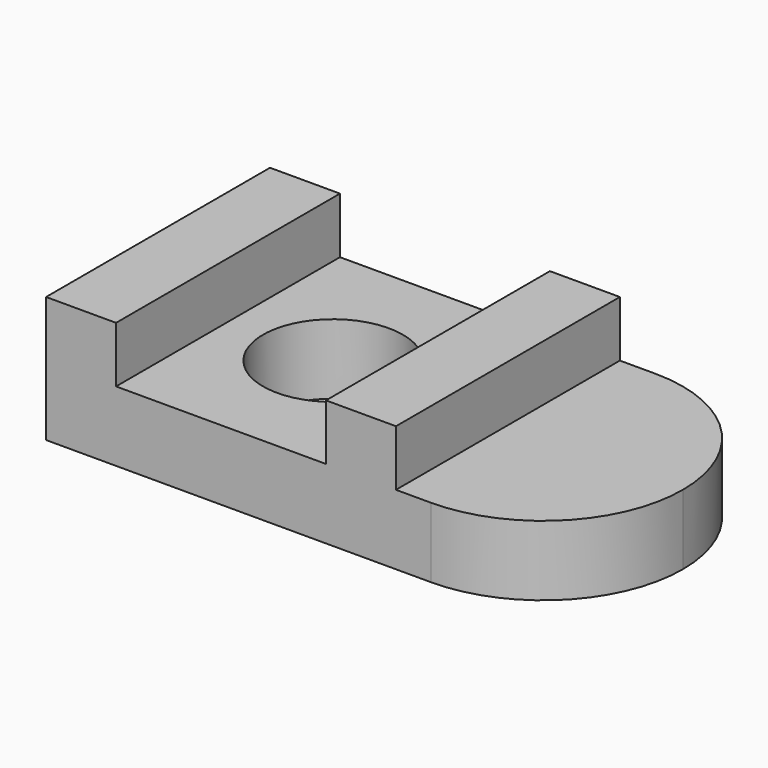
from build123d import *

# Parameters (mm, degrees)
F1_DEPTH = 40
F2_R     = 19.99999
F3_R     = 10
F4_DEPTH = 10


# Not quite as in the source:
# - a fillet or chamfer is up to 0.001 mm smaller than in the source, because OpenCascade refuses the exact size


with BuildPart() as f1:
    # F0 (on Front) → F1 (new body)
    with BuildSketch(Plane.XZ):
        Polygon((0, 18), (0, 0), (75, 0), (75, 10), (50, 10), (50, 18), (40, 18), (40, 10), (10, 10), (10, 18), align=None)
    extrude(amount=F1_DEPTH)

    # F2 (radius 20 in the source; OpenCascade refuses exactly that, so slightly less here)
    f2_edges = [f1.edges().sort_by_distance(p)[0] for p in [
        (75, -40, 5),
        (75, 0, 5),
    ]]
    fillet(f2_edges, radius=F2_R)

    # F3 (on face) → F4 (cut, through all)
    with BuildSketch(Plane.XY.offset(10)):
        with Locations((25, -20)):
            Circle(F3_R)
    extrude(amount=-F4_DEPTH, mode=Mode.SUBTRACT)


solid = f1.part
